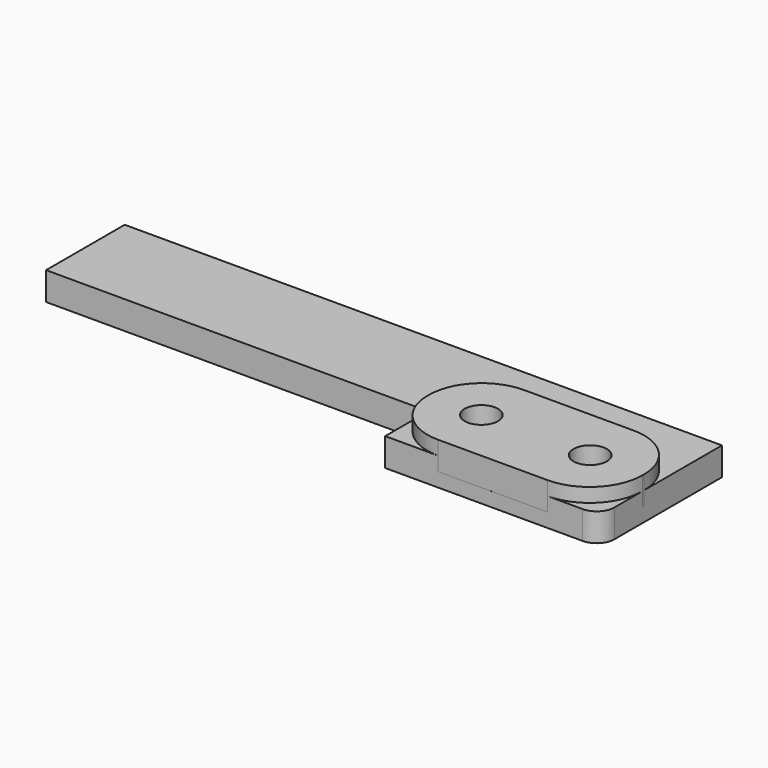
from build123d import *

# Parameters (mm, degrees)
F0_W     = 30.6375
F0_H     = 30.6375
F0_R     = 10.31875
F0_W_2   = 15.1375
F0_H_2   = 12.68125
F1_DEPTH = 4
F2_DEPTH = 8
F3_D     = 9.525
F4_R     = 15
F5_R     = 5


# Not quite as in the source:
# - a length typed as a fraction of an inch, garbled in the dataset ("3 / 203.2 mm" for 3/8 in), is restored


with BuildPart() as f1:
    # F0 (on Top) → F1 (new body, symmetric)
    with BuildSketch(Plane.XY):
        with BuildLine():
            Line((-30.6375, -15.31875), (0, -15.31875))
            Line((0, -15.31875), (0, 15.31875))
            Line((0, 15.31875), (-15.5, 15.31875))
            Line((-15.5, 15.31875), (-15.5, 10.31875))
            ThreePointArc((-15.5, 10.31875), (-8.2035419016, 7.2964580984), (-5.18125, 0))
            ThreePointArc((-5.18125, 0), (-15.5, -10.31875), (-25.81875, 0))
            Line((-25.81875, 0), (-30.6375, 0))
            Line((-30.6375, 0), (-30.6375, -15.31875))
        make_face()
        with BuildLine():
            Line((-30.6375, 15.31875), (-30.6375, 0))
            Line((-30.6375, 0), (-25.81875, 0))
            ThreePointArc((-25.81875, 0), (-22.7964580984, 7.2964580984), (-15.5, 10.31875))
            Line((-15.5, 10.31875), (-15.5, 15.31875))
            Line((-15.5, 15.31875), (-30.6375, 15.31875))
        make_face()
        with Locations((15.31875, 0)):
            Rectangle(F0_W, F0_H)
        with Locations((15.5, 0)):
            Circle(F0_R, mode=Mode.SUBTRACT)
        with BuildLine():
            Line((-30.6375, -15.31875), (0, -15.31875))
            Line((0, -15.31875), (0, 15.31875))
            Line((0, 15.31875), (-15.5, 15.31875))
            Line((-15.5, 15.31875), (-15.5, 10.31875))
            ThreePointArc((-15.5, 10.31875), (-8.2035419016, 7.2964580984), (-5.18125, 0))
            ThreePointArc((-5.18125, 0), (-15.5, -10.31875), (-25.81875, 0))
            Line((-25.81875, 0), (-30.6375, 0))
            Line((-30.6375, 0), (-30.6375, -15.31875))
        make_face()
        Polygon((0, 15.31875), (30.6375, 15.31875), (30.6375, 28), (-15.5, 28), (-15.5, 15.31875), align=None)
        with Locations((-23.06875, 21.659375)):
            Rectangle(F0_W_2, F0_H_2)
        Polygon((-139.5, 0), (-30.6375, 0), (-30.6375, 15.31875), (-30.6375, 28), (-139.5, 28), align=None)
    extrude(amount=F1_DEPTH, both=True)

    # F5
    f5_edges = [f1.edges().sort_by_distance(p)[0] for p in [
        (30.6375, -15.31875, 0),
    ]]
    fillet(f5_edges, radius=F5_R)


with BuildPart() as f2:
    # F0 (on Top) → F2 (new body)
    with BuildSketch(Plane.XY):
        with BuildLine():
            Line((-30.6375, -15.31875), (0, -15.31875))
            Line((0, -15.31875), (0, 15.31875))
            Line((0, 15.31875), (-15.5, 15.31875))
            Line((-15.5, 15.31875), (-15.5, 10.31875))
            ThreePointArc((-15.5, 10.31875), (-8.2035419016, 7.2964580984), (-5.18125, 0))
            ThreePointArc((-5.18125, 0), (-15.5, -10.31875), (-25.81875, 0))
            Line((-25.81875, 0), (-30.6375, 0))
            Line((-30.6375, 0), (-30.6375, -15.31875))
        make_face()
        with BuildLine():
            Line((-30.6375, 15.31875), (-30.6375, 0))
            Line((-30.6375, 0), (-25.81875, 0))
            ThreePointArc((-25.81875, 0), (-22.7964580984, 7.2964580984), (-15.5, 10.31875))
            Line((-15.5, 10.31875), (-15.5, 15.31875))
            Line((-15.5, 15.31875), (-30.6375, 15.31875))
        make_face()
        with BuildLine():
            Line((-30.6375, -15.31875), (0, -15.31875))
            Line((0, -15.31875), (0, 15.31875))
            Line((0, 15.31875), (-15.5, 15.31875))
            Line((-15.5, 15.31875), (-15.5, 10.31875))
            ThreePointArc((-15.5, 10.31875), (-8.2035419016, 7.2964580984), (-5.18125, 0))
            ThreePointArc((-5.18125, 0), (-15.5, -10.31875), (-25.81875, 0))
            Line((-25.81875, 0), (-30.6375, 0))
            Line((-30.6375, 0), (-30.6375, -15.31875))
        make_face()
        with Locations((15.31875, 0)):
            Rectangle(F0_W, F0_H)
        with Locations((15.5, 0)):
            Circle(F0_R, mode=Mode.SUBTRACT)
        with Locations((15.5, 0)):
            Circle(F0_R)
        with BuildLine():
            Line((-15.5, 0), (-25.81875, 0))
            ThreePointArc((-25.81875, 0), (-15.5, -10.31875), (-5.18125, 0))
            ThreePointArc((-5.18125, 0), (-8.2035419016, 7.2964580984), (-15.5, 10.31875))
            Line((-15.5, 10.31875), (-15.5, 0))
        make_face()
        with BuildLine():
            ThreePointArc((-15.5, 10.31875), (-22.7964580984, 7.2964580984), (-25.81875, 0))
            Line((-25.81875, 0), (-15.5, 0))
            Line((-15.5, 0), (-15.5, 10.31875))
        make_face()
    extrude(amount=F2_DEPTH)

    # F3 (through all)
    with Locations(Plane(origin=(0, 0, 0), x_dir=(1, 0, 0), z_dir=(0, 0, -1))):
        with Locations((-15.5, 0), (15.5, 0)):
            Hole(F3_D / 2)

    # F4
    f4_edges = [f2.edges().sort_by_distance(p)[0] for p in [
        (30.6375, 15.31875, 4),
        (30.6375, -15.31875, 4),
        (-30.6375, -15.31875, 4),
        (-30.6375, 15.31875, 4),
    ]]
    fillet(f4_edges, radius=F4_R)


solid = Compound([f1.part, f2.part])
